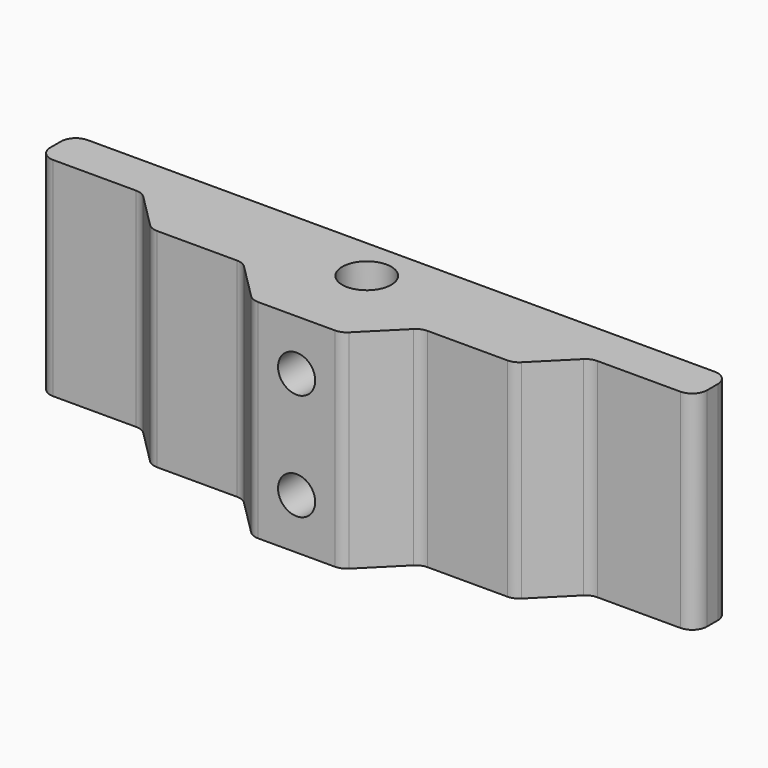
from build123d import *

# Parameters (mm, degrees)
F0_W         = 7.62
F0_H         = 3.81
F1_DEPTH     = 17.78
F2_W         = 51.562
F2_H         = 1.143
F2_W_2       = 26.162
F3_DEPTH     = 7.62
F4_T4_DEPTH  = 17.78
F4_T9_DEPTH  = 17.78
F4_T14_DEPTH = 17.78
F4_T19_DEPTH = 17.78
F5_R         = 1.5875
F6_DEPTH     = 25.4
F7_R         = 2.0955
F8_DEPTH     = 7.62
F9_R         = 1.27


# Not quite as in the source:
# - a fillet or chamfer that OpenCascade refuses, or shapes differently, is made with other operations: its cross-section is extruded or revolved along the edge and cut away or added


with BuildPart() as f1:
    # F0 (on Top) → F1 (new body)
    with BuildSketch(Plane.XY):
        Polygon((0, 3.683), (0, 0), (12.7, 0), (43.434, 0), (56.134, 0), (56.134, 3.683), align=None)
        Polygon((43.434, 0), (12.7, 0), (12.7, -3.683), (24.257, -3.683), (31.877, -3.683), (43.434, -3.683), align=None)
        with Locations((28.067, -5.588)):
            Rectangle(F0_W, F0_H)
    extrude(amount=F1_DEPTH)

    # F2 (on face) → F3 (cut)
    with BuildSketch(Plane(origin=(0, 0, 0), x_dir=(1, 0, 0), z_dir=(0, 0, -1))):
        with Locations((28.067, -1.8415)):
            Rectangle(F2_W, F2_H)
        with Locations((28.067, 1.8415)):
            Rectangle(F2_W_2, F2_H)
    extrude(amount=-F3_DEPTH, mode=Mode.SUBTRACT)

    # F4: chamfer of 3.81 on 4 edges, made by hand


with BuildPart() as f4_tool2:
    # F4_s3 → F4_t4 (new body)
    with BuildSketch(Plane.XY):
        Polygon((35.687, -3.683), (31.877, -7.493), (31.877, -3.683), align=None)
    extrude(amount=F4_T4_DEPTH)

    split(bisect_by=Plane.XZ.offset(7.493), keep=Keep.BOTTOM)


with BuildPart() as f1_1:
    add(f1.part)

    # F4_t1: union F4_tool2
    add(f4_tool2.part)


with BuildPart() as f4_tool7:
    # F4_s8 → F4_t9 (new body)
    with BuildSketch(Plane.XY):
        Polygon((47.244, 0), (43.434, -3.81), (43.434, 0), align=None)
    extrude(amount=F4_T9_DEPTH)

    split(bisect_by=Plane.XZ.offset(3.683), keep=Keep.BOTTOM)


with BuildPart() as f1_2:
    add(f1_1.part)

    # F4_t6: union F4_tool7
    add(f4_tool7.part)


with BuildPart() as f4_tool12:
    # F4_s13 → F4_t14 (new body)
    with BuildSketch(Plane.XY):
        Polygon((20.447, -3.683), (24.257, -7.493), (24.257, -3.683), align=None)
    extrude(amount=F4_T14_DEPTH)

    split(bisect_by=Plane.XZ.offset(7.493), keep=Keep.BOTTOM)


with BuildPart() as f1_3:
    add(f1_2.part)

    # F4_t11: union F4_tool12
    add(f4_tool12.part)


with BuildPart() as f4_tool17:
    # F4_s18 → F4_t19 (new body)
    with BuildSketch(Plane.XY):
        Polygon((8.89, 0), (12.7, -3.81), (12.7, 0), align=None)
    extrude(amount=F4_T19_DEPTH)

    split(bisect_by=Plane.XZ.offset(3.683), keep=Keep.BOTTOM)


with BuildPart() as f1_4:
    add(f1_3.part)

    # F4_t16: union F4_tool17
    add(f4_tool17.part)

    # F5 (on face) → F6 (cut)
    with BuildSketch(Plane.XZ.offset(7.493)):
        with Locations((28.067, 13.462)):
            Circle(F5_R)
        with Locations((28.067, 4.318)):
            Circle(F5_R)
    extrude(amount=-F6_DEPTH, mode=Mode.SUBTRACT)

    # F7 (on face) → F8 (cut)
    with BuildSketch(Plane.XY.offset(17.78)):
        with Locations((28.067, 0)):
            Circle(F7_R)
    extrude(amount=-F8_DEPTH, mode=Mode.SUBTRACT)

    # F9
    f9_edges = [f1_4.edges().sort_by_distance(p)[0] for p in [
        (0, 0, 8.89),
        (56.134, 0, 8.89),
        (56.134, 3.683, 8.89),
        (0, 3.683, 8.89),
        (12.573, -3.683, 8.89),
        (43.561, -3.683, 8.89),
        (31.877, -7.493, 8.89),
        (24.257, -7.493, 8.89),
        (8.89, 0, 8.89),
        (47.244, 0, 8.89),
        (35.687, -3.683, 8.89),
        (20.447, -3.683, 8.89),
    ]]
    fillet(f9_edges, radius=F9_R)


solid = f1_4.part
